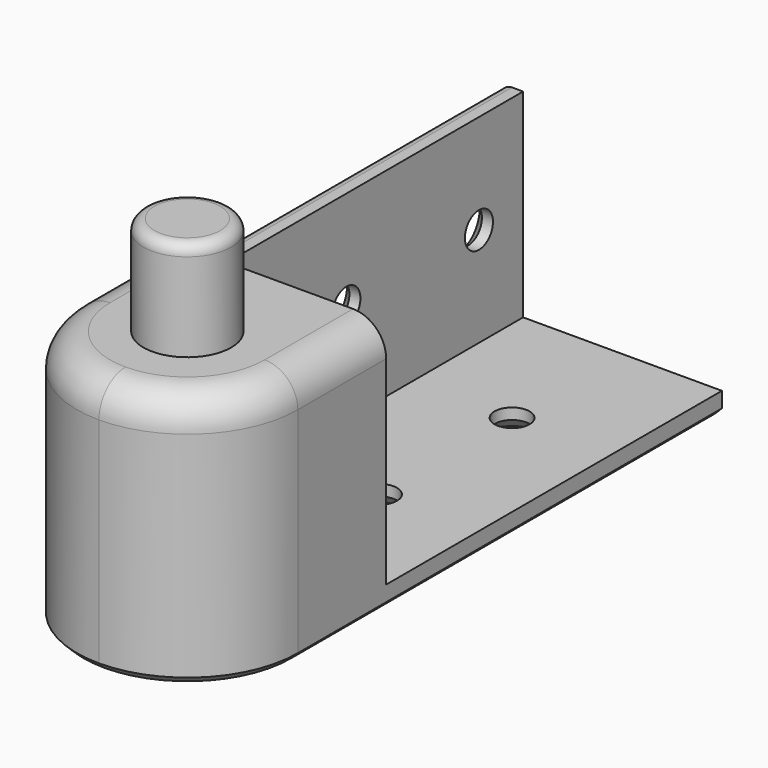
from build123d import *

# Parameters (mm, degrees)
F1_DEPTH     = 40
F2_W         = 2
F2_H         = 18
F3_DEPTH     = 18
F4_R         = 1.5875
F5_DEPTH     = 2.001
F6_R         = 1.5875
F7_DEPTH     = 2.001
F8_SIZE      = 1
F9_W         = 20
F9_H         = 18
F10_DEPTH    = 20
F12_DEPTH    = 3
F13_R        = 3.975
F14_DEPTH    = 9
F15_R        = 1
F16_R        = 9.99999
F17_R        = 3
F18_T1_DEPTH = 40.5
F19_SIZE     = 0.6


# Not quite as in the source:
# - a fillet or chamfer that OpenCascade refuses, or shapes differently, is made with other operations: its cross-section is extruded or revolved along the edge and cut away or added
# - a fillet or chamfer is up to 0.001 mm smaller than in the source, because OpenCascade refuses the exact size


with BuildPart() as f1:
    # F0 (on Front) → F1 (new body)
    with BuildSketch(Plane.XZ):
        Polygon((-2, 18), (-2, -2), (18, -2), (18, 0), (0, 0), (0, 18), align=None)
    extrude(amount=-F1_DEPTH)

    # F2 (on face) → F3 (join, through all)
    with BuildSketch(Plane.YZ):
        with Locations((1, 9)):
            Rectangle(F2_W, F2_H)
    extrude(amount=F3_DEPTH)

    # F4 (on face) → F5 (cut, through all)
    with BuildSketch(Plane.XY):
        with Locations((9, 12.5)):
            Circle(F4_R)
        with Locations((9, 27.5)):
            Circle(F4_R)
    extrude(amount=-F5_DEPTH, mode=Mode.SUBTRACT)

    # F6 (on face) → F7 (cut, through all)
    with BuildSketch(Plane.YZ):
        with Locations((35, 9)):
            Circle(F6_R)
        with Locations((20, 9)):
            Circle(F6_R)
    extrude(amount=-F7_DEPTH, mode=Mode.SUBTRACT)

    # F8
    f8_edges = [f1.edges().sort_by_distance(p)[0] for p in [
        (-2, 18.4125, 9),
        (-2, 33.4125, 9),
        (7.4125, 27.5, -2),
        (7.4125, 12.5, -2),
    ]]
    chamfer(f8_edges, length=F8_SIZE)

    # F9 (on face) → F10 (join, through all)
    with BuildSketch(Plane.XY.offset(18)):
        with Locations((8, -9)):
            Rectangle(F9_W, F9_H)
    extrude(amount=-F10_DEPTH)

    # F11 (on face) → F12 (join)
    with BuildSketch(Plane.XY.offset(18)):
        Polygon((18, -18), (18, 2), (0, 2), (-2, 2), (-2, -18), align=None)
    extrude(amount=F12_DEPTH)

    # F13 (on face) → F14 (join)
    with BuildSketch(Plane.XY.offset(21)):
        with Locations((8, -8)):
            Circle(F13_R)
    extrude(amount=F14_DEPTH)

    # F15
    f15_edges = [f1.edges().sort_by_distance(p)[0] for p in [
        (4.025, -8, 30),
    ]]
    fillet(f15_edges, radius=F15_R)

    # F16 (radius 10 in the source; OpenCascade refuses exactly that, so slightly less here)
    f16_edges = [f1.edges().sort_by_distance(p)[0] for p in [
        (-2, -18, 9.5),
        (18, -18, 9.5),
    ]]
    fillet(f16_edges, radius=F16_R)

    # F17
    f17_edges = [f1.edges().sort_by_distance(p)[0] for p in [
        (0.928929, -15.071071, 21),
        (-2, -3.000005, 21),
        (18, -3.000005, 21),
        (15.071071, -15.071071, 21),
        (8, -18, 21),
    ]]
    fillet(f17_edges, radius=F17_R)

    # F18: fillet of radius 1 on 1 edges, made by hand

    # F18_s2 → F18_t1 (cut)
    with BuildSketch(Plane.XZ.offset(-42.5)):
        with BuildLine():
            ThreePointArc((-1, 18), (-1.7071067812, 17.7071067812), (-2, 17))
            Line((-2, 17), (-2, 18))
            Line((-2, 18), (-1, 18))
        make_face()
    extrude(amount=F18_T1_DEPTH, mode=Mode.SUBTRACT)

    # F19
    f19_edges = [f1.edges().sort_by_distance(p)[0] for p in [
        (18, 15.999995, -2),
        (-2, 15.999995, -2),
        (0.928929, -15.071071, -2),
        (15.071071, -15.071071, -2),
        (8, -18, -2),
    ]]
    chamfer(f19_edges, length=F19_SIZE)


solid = f1.part
